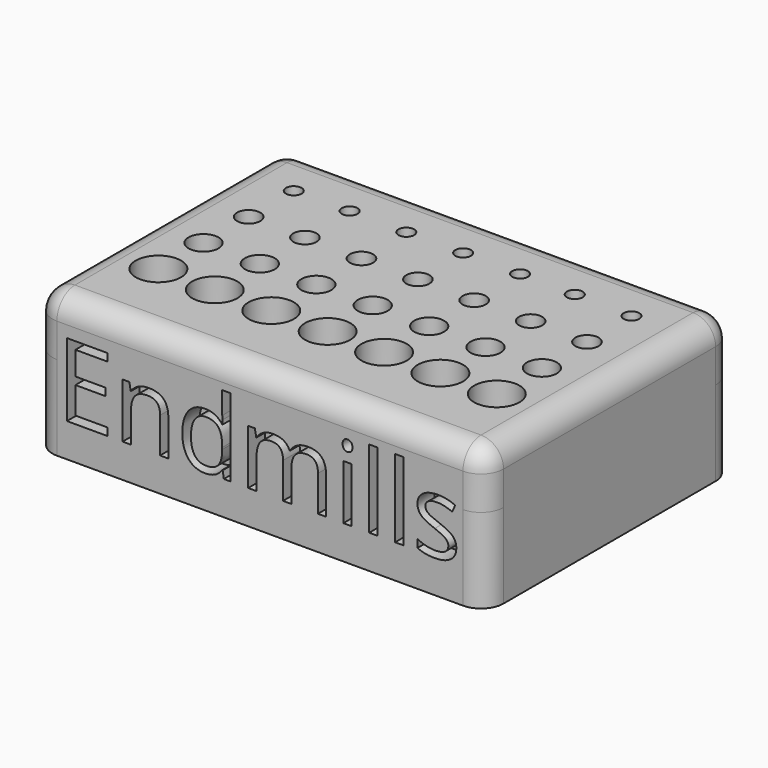
from build123d import *

# Parameters (mm, degrees)
F0_W         = 101.6
F0_H         = 69.85
F1_DEPTH     = 19.05
F2_R         = 5.08
F3_R         = 5.08
F4_R         = 5.0998793322
F4_R_2       = 3.3685858291
F4_R_3       = 2.6085039477
F4_R_4       = 1.7674524104
F5_DEPTH     = 12.7
F6_R         = 5.08
F7_TEXT_SIZE = 23.0463513567
F8_DEPTH     = 4.7625


# Not quite as in the source:
# - Text() gives the source's letters only with a copy of the font that has no kerning and outlines rounded to 1/6400 em; it was checked with that copy


with BuildPart() as f1:
    # F0 (on Top) → F1 (new body)
    with BuildSketch(Plane.XY):
        with Locations((50.8, -34.925)):
            Rectangle(F0_W, F0_H)
    extrude(amount=F1_DEPTH)

    # F2
    f2_edges = [f1.edges().sort_by_distance(p)[0] for p in [
        (101.6, -69.85, 9.525),
        (0, -69.85, 9.525),
    ]]
    fillet(f2_edges, radius=F2_R)

    # F3
    f3_edges = [f1.edges().sort_by_distance(p)[0] for p in [
        (0, 0, 9.525),
        (101.6, 0, 9.525),
    ]]
    fillet(f3_edges, radius=F3_R)

    # F4 (on face) → F5 (join)
    with BuildSketch(Plane.XY.offset(19.05)):
        with BuildLine():
            ThreePointArc((5.08, 0), (1.4878975516, -1.4878975516), (0, -5.08))
            Line((0, -5.08), (0, -64.77))
            ThreePointArc((0, -64.77), (1.4878975516, -68.3621024484), (5.08, -69.85))
            Line((5.08, -69.85), (96.52, -69.85))
            ThreePointArc((96.52, -69.85), (100.1121024484, -68.3621024484), (101.6, -64.77))
            Line((101.6, -64.77), (101.6, -5.08))
            ThreePointArc((101.6, -5.08), (100.1121024484, -1.4878975516), (96.52, 0))
            Line((96.52, 0), (5.08, 0))
        make_face()
        with Locations((12.7, -50.8)):
            Circle(F4_R, mode=Mode.SUBTRACT)
        with Locations((12.7, -38.1)):
            Circle(F4_R_2, mode=Mode.SUBTRACT)
        with Locations((25.3887362778, -38.1193496287)):
            Circle(F4_R_2, mode=Mode.SUBTRACT)
        with Locations((25.4101790488, -50.81795156)):
            Circle(F4_R, mode=Mode.SUBTRACT)
        with Locations((38.1118059158, -50.8031845093)):
            Circle(F4_R, mode=Mode.SUBTRACT)
        with Locations((38.1040908396, -38.1003469229)):
            Circle(F4_R_2, mode=Mode.SUBTRACT)
        with Locations((50.8134327829, -50.8031845093)):
            Circle(F4_R, mode=Mode.SUBTRACT)
        with Locations((63.5150596499, -50.7884174585)):
            Circle(F4_R, mode=Mode.SUBTRACT)
        with Locations((50.8004426956, -38.1003469229)):
            Circle(F4_R_2, mode=Mode.SUBTRACT)
        with Locations((63.5157972574, -38.1003431976)):
            Circle(F4_R_2, mode=Mode.SUBTRACT)
        with Locations((76.201915741, -50.8031882346)):
            Circle(F4_R, mode=Mode.SUBTRACT)
        with Locations((88.9035537839, -50.8031882346)):
            Circle(F4_R, mode=Mode.SUBTRACT)
        with Locations((76.2311518192, -38.1383560598)):
            Circle(F4_R_2, mode=Mode.SUBTRACT)
        with Locations((88.9084935188, -38.1193496287)):
            Circle(F4_R_2, mode=Mode.SUBTRACT)
        with Locations((12.7, -25.4)):
            Circle(F4_R_3, mode=Mode.SUBTRACT)
        with Locations((25.3694262356, -25.3934822977)):
            Circle(F4_R_3, mode=Mode.SUBTRACT)
        with Locations((38.0946062505, -25.3884736449)):
            Circle(F4_R_3, mode=Mode.SUBTRACT)
        with Locations((12.7, -12.7)):
            Circle(F4_R_4, mode=Mode.SUBTRACT)
        with Locations((25.1819584519, -12.5715378672)):
            Circle(F4_R_4, mode=Mode.SUBTRACT)
        with Locations((38.0016118288, -12.6581573859)):
            Circle(F4_R_4, mode=Mode.SUBTRACT)
        with Locations((50.7346428931, -12.5715378672)):
            Circle(F4_R_4, mode=Mode.SUBTRACT)
        with Locations((50.8092828095, -25.4047121853)):
            Circle(F4_R_3, mode=Mode.SUBTRACT)
        with Locations((63.4961649776, -25.4194773734)):
            Circle(F4_R_3, mode=Mode.SUBTRACT)
        with Locations((76.2189850211, -25.4194773734)):
            Circle(F4_R_3, mode=Mode.SUBTRACT)
        with Locations((88.9049768448, -25.4194773734)):
            Circle(F4_R_3, mode=Mode.SUBTRACT)
        with Locations((63.5542944074, -12.5715378672)):
            Circle(F4_R_4, mode=Mode.SUBTRACT)
        with Locations((75.9408473969, -12.6581573859)):
            Circle(F4_R_4, mode=Mode.SUBTRACT)
        with Locations((88.8471230865, -12.831395492)):
            Circle(F4_R_4, mode=Mode.SUBTRACT)
    extrude(amount=F5_DEPTH)

    # F6
    f6_edges = [f1.edges().sort_by_distance(p)[0] for p in [
        (50.8, -69.85, 31.75),
    ]]
    fillet(f6_edges, radius=F6_R)

    # F7 (on face) → F8 (cut)
    with BuildSketch(Plane.XZ.offset(69.85)):
        with Locations((5.08, 7.5912453642)):
            Text('Endmills', F7_TEXT_SIZE, font='Open Sans', text_align=(TextAlign.LEFT, TextAlign.BOTTOM))
    extrude(amount=-F8_DEPTH, mode=Mode.SUBTRACT)


solid = f1.part
